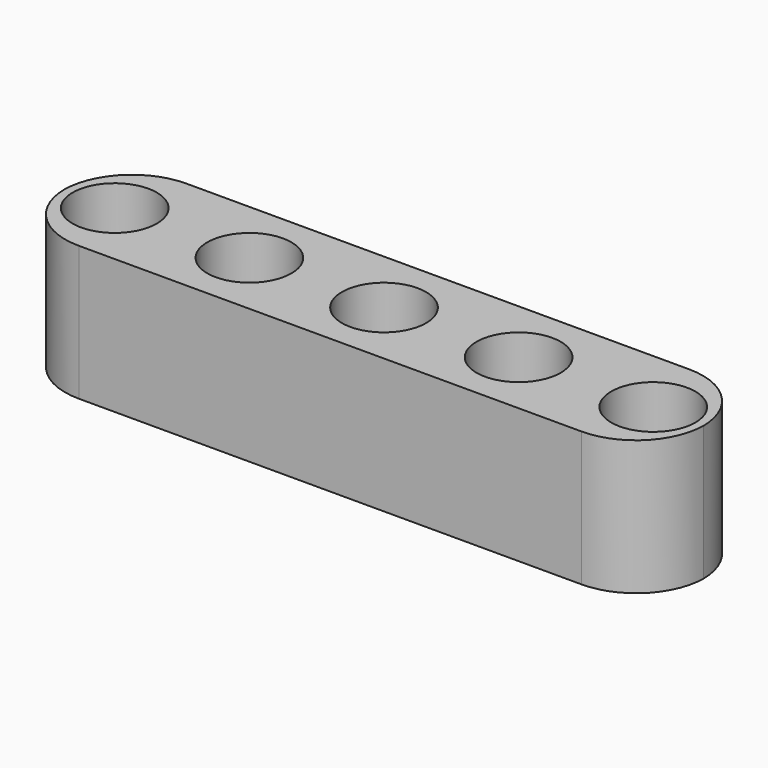
from build123d import *

# Parameters (mm, degrees)
F0_W        = 38
F0_H        = 8
F0_R        = 2.5
F1_DEPTH    = 8
F2_T1_DEPTH = 28.32


# Not quite as in the source:
# - a fillet or chamfer that OpenCascade refuses, or shapes differently, is made with other operations: its cross-section is extruded or revolved along the edge and cut away or added


with BuildPart() as f1:
    # F0 (on Top) → F1 (new body)
    with BuildSketch(Plane.XY):
        Rectangle(F0_W, F0_H)
        with BuildLine():
            ThreePointArc((-18.5, 0), (-16, 2.5), (-13.5, 0))
            ThreePointArc((-13.5, 0), (-16, -2.5), (-18.5, 0))
        make_face(mode=Mode.SUBTRACT)
        with Locations((-8, 0)):
            Circle(F0_R, mode=Mode.SUBTRACT)
        Circle(F0_R, mode=Mode.SUBTRACT)
        with Locations((8, 0)):
            Circle(F0_R, mode=Mode.SUBTRACT)
        with Locations((16, 0)):
            Circle(F0_R, mode=Mode.SUBTRACT)
    extrude(amount=F1_DEPTH)

    # F2: fillet of radius 4.064 on 4 edges, made by hand

    # F2_s2 → F2_t1 (cut)
    with BuildSketch(Plane.XY.offset(-10.16)):
        with BuildLine():
            ThreePointArc((14.936, -4), (17.8096819587, -2.8096819587), (19, 0.064))
            Line((19, 0.064), (19, -4))
            Line((19, -4), (14.936, -4))
        make_face()
        with BuildLine():
            ThreePointArc((14.936, 4), (17.8096819587, 2.8096819587), (19, -0.064))
            Line((19, -0.064), (19, 4))
            Line((19, 4), (14.936, 4))
        make_face()
        with BuildLine():
            ThreePointArc((-14.936, -4), (-17.8096819587, -2.8096819587), (-19, 0.064))
            Line((-19, 0.064), (-19, -4))
            Line((-19, -4), (-14.936, -4))
        make_face()
        with BuildLine():
            ThreePointArc((-14.936, 4), (-17.8096819587, 2.8096819587), (-19, -0.064))
            Line((-19, -0.064), (-19, 4))
            Line((-19, 4), (-14.936, 4))
        make_face()
    extrude(amount=F2_T1_DEPTH, mode=Mode.SUBTRACT)


solid = f1.part
